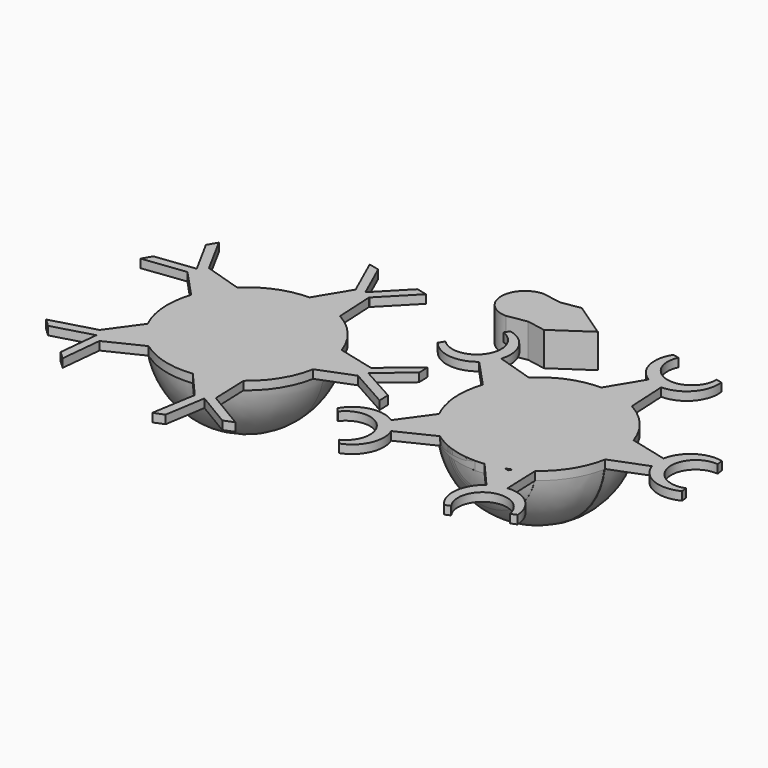
from build123d import *

# Parameters (mm, degrees)
F3_DEPTH = 1.27
F4_ANGLE = 180
F5_ANGLE = 180
F6_DEPTH = 5.08


# Not quite as in the source:
# - a feature names something its author has since deleted; it is built from what else it names


with BuildPart() as f3:
    # F0 (on Top) → F3 (new body)
    with BuildSketch(Plane.XY):
        with BuildLine():
            Line((4.8936784242, -7.1238775551), (4.5592080627, -7.6555667928))
            Line((4.5592080627, -7.6555667928), (3.9454245804, -7.5005655384))
            ThreePointArc((3.9454245804, -7.5005655384), (2.6783186026, -7.8645703011), (1.3787031683, -8.086057883))
            Line((1.3787031683, -8.086057883), (4.9129540048, -12.1410587354))
            Line((4.9129540048, -12.1410587354), (4.9601170844, -12.1951710033))
            Line((4.9601170844, -12.1951710033), (6.1814893534, -11.7059845827))
            Line((6.1814893534, -11.7059845827), (7.3584312348, -11.2345935081))
            Line((7.3584312348, -11.2345935081), (7.1565504338, -5.792935627))
            ThreePointArc((7.1565504338, -5.792935627), (6.061960316, -6.5210520939), (4.8936784242, -7.1238775551))
        make_face()
        with BuildLine():
            ThreePointArc((1.3787031683, -8.086057883), (2.6783186026, -7.8645703011), (3.9454245804, -7.5005655384))
            ThreePointArc((3.9454245804, -7.5005655384), (4.1864101627, -7.4136951085), (4.4254683384, -7.3216532098))
            ThreePointArc((4.4254683384, -7.3216532098), (4.6606303031, -7.2252675178), (4.8936784242, -7.1238775551))
            ThreePointArc((4.8936784242, -7.1238775551), (6.061960316, -6.5210520939), (7.1565504338, -5.792935627))
            Line((7.1565504338, -5.792935627), (7.1556255471, -5.7680054855))
            ThreePointArc((7.1556255471, -5.7680054855), (10.1274372954, -2.5017266103), (11.7022892851, 1.6238138354))
            Line((11.7022892851, 1.6238138354), (11.7389820542, 1.6381275484))
            ThreePointArc((11.7389820542, 1.6381275484), (11.8913668028, 4.6083597915), (11.3018507931, 7.5234878441))
            Line((11.3018507931, 7.5234878441), (11.2645029558, 7.5329194463))
            ThreePointArc((11.2645029558, 7.5329194463), (9.1157339139, 11.3612670795), (5.7241812928, 14.1488869988))
            Line((5.7241812928, 14.1488869988), (5.7231708963, 14.1682476177))
            ThreePointArc((5.7231708963, 14.1682476177), (2.9312146583, 15.2592925332), (-0.0448824936, 15.6174047842))
            Line((-0.0448824936, 15.6174047842), (0, -8.1622908183))
            ThreePointArc((0, -8.1622908183), (0.6889378263, -8.1423144191), (1.3755606611, -8.0824523468))
            Line((1.3755606611, -8.0824523468), (1.3787031683, -8.086057883))
        make_face()
        with BuildLine():
            ThreePointArc((0, -8.1622908183), (0.6904591534, -8.1442051837), (1.3787031683, -8.086057883))
            Line((1.3787031683, -8.086057883), (1.3755606611, -8.0824523468))
            ThreePointArc((1.3755606611, -8.0824523468), (0.6889378263, -8.1423144191), (0, -8.1622908183))
        make_face()
        with BuildLine():
            Line((7.1556255471, -5.7680054855), (7.1565504338, -5.792935627))
            ThreePointArc((7.1565504338, -5.792935627), (10.1544844582, -2.5132081517), (11.7389820542, 1.6381275484))
            Line((11.7389820542, 1.6381275484), (11.7022892851, 1.6238138354))
            ThreePointArc((11.7022892851, 1.6238138354), (10.1274372954, -2.5017266103), (7.1556255471, -5.7680054855))
        make_face()
        with BuildLine():
            Line((4.9601170844, -12.1951710033), (4.9129540048, -12.1410587354))
            ThreePointArc((4.9129540048, -12.1410587354), (2.9744543706, -15.5193953097), (4.1887523177, -19.2202626859))
            Line((4.1887523177, -19.2202626859), (5.0008226603, -18.8854850019))
            ThreePointArc((5.0008226603, -18.8854850019), (6.5893352056, -13.3433475455), (11.622070306, -16.1558619191))
            Line((11.622070306, -16.1558619191), (12.518363314, -15.7863632665))
            ThreePointArc((12.518363314, -15.7863632665), (10.9032070899, -12.4167602553), (7.3584312348, -11.2345935081))
            Line((7.3584312348, -11.2345935081), (6.1814893534, -11.7059845827))
            Line((6.1814893534, -11.7059845827), (4.9601170844, -12.1951710033))
        make_face()
        with BuildLine():
            ThreePointArc((-7.0516919086, -5.8454424545), (-3.7112715178, -7.5682384641), (0, -8.1622908183))
            Line((0, -8.1622908183), (-0.0448824936, 15.6174047842))
            ThreePointArc((-0.0448824936, 15.6174047842), (-4.4734734608, 14.743838405), (-8.2573042209, 12.2825052394))
            Line((-8.2573042209, 12.2825052394), (-13.7991155098, 14.0226887463))
            Line((-13.7991155098, 14.0226887463), (-13.8825975476, 14.0489029311))
            Line((-13.8825975476, 14.0489029311), (-14.5983996738, 12.9110314466))
            Line((-14.5983996738, 12.9110314466), (-15.319207147, 11.7652032356))
            Line((-15.319207147, 11.7652032356), (-11.2936160838, 7.4456261961))
            ThreePointArc((-11.2936160838, 7.4456261961), (-11.8627160209, 2.9241962242), (-10.6891807971, -1.4792136827))
            Line((-10.6891807971, -1.4792136827), (-14.1287515965, -6.2587273525))
            Line((-14.1287515965, -6.2587273525), (-14.1557744366, -6.2962773961))
            Line((-14.1557744366, -6.2962773961), (-13.2794303468, -7.3470839927))
            Line((-13.2794303468, -7.3470839927), (-12.3756340088, -8.4308080287))
            Line((-12.3756340088, -8.4308080287), (-7.0516919086, -5.8454424545))
        make_face()
        with BuildLine():
            ThreePointArc((11.3018507931, 7.5234878441), (11.8913668028, 4.6083597915), (11.7389820542, 1.6381275484))
            Line((11.7389820542, 1.6381275484), (17.0952796063, 3.7275993392))
            Line((17.0952796063, 3.7275993392), (17.0191165937, 4.8661190757))
            Line((17.0191165937, 4.8661190757), (16.936538316, 6.1005371469))
            Line((16.936538316, 6.1005371469), (11.3018507931, 7.5234878441))
        make_face()
        with BuildLine():
            Line((3.0023803732, 20.6531485623), (-0.0448824936, 15.6174047842))
            ThreePointArc((-0.0448824936, 15.6174047842), (2.9312146583, 15.2592925332), (5.7231708963, 14.1682476177))
            Line((5.7231708963, 14.1682476177), (5.4165524673, 20.0434878046))
            Line((5.4165524673, 20.0434878046), (5.4515073631, 20.0616481273))
            ThreePointArc((5.4515073631, 20.0616481273), (9.0104590154, 21.6991770677), (10.1547438103, 25.4459423662))
            Line((10.1547438103, 25.4459423662), (9.2975141381, 25.6374929551))
            ThreePointArc((9.2975141381, 25.6374929551), (4.8174413872, 22.0087730928), (2.308058113, 27.1993082555))
            Line((2.308058113, 27.1993082555), (1.3619221427, 27.4107252283))
            ThreePointArc((1.3619221427, 27.4107252283), (0.7522557785, 23.7240924821), (2.9779031767, 20.7225182718))
            Line((2.9779031767, 20.7225182718), (3.0023803732, 20.6531485623))
        make_face()
        with BuildLine():
            Line((17.0191165937, 4.8661190757), (17.0952796063, 3.7275993392))
            Line((17.0952796063, 3.7275993392), (17.1615459763, 3.5500786447))
            ThreePointArc((17.1615459763, 3.5500786447), (19.9175529921, 0.7658259222), (23.8297291445, 0.9720191488))
            Line((23.8297291445, 0.9720191488), (23.7165380041, 1.8430657059))
            ThreePointArc((23.7165380041, 1.8430657059), (18.7743816021, 4.8118617231), (22.7936295654, 8.9451782489))
            Line((22.7936295654, 8.9451782489), (22.6686989745, 9.9065641017))
            ThreePointArc((22.6686989745, 9.9065641017), (18.99587921, 9.2185604251), (16.936538316, 6.1005371469))
            Line((16.936538316, 6.1005371469), (17.0191165937, 4.8661190757))
        make_face()
        with BuildLine():
            Line((11.2645029558, 7.5329194463), (11.3018507931, 7.5234878441))
            ThreePointArc((11.3018507931, 7.5234878441), (9.1402278714, 11.3728743462), (5.7231708963, 14.1682476177))
            Line((5.7231708963, 14.1682476177), (5.7241812928, 14.1488869988))
            ThreePointArc((5.7241812928, 14.1488869988), (9.1157339139, 11.3612670795), (11.2645029558, 7.5329194463))
        make_face()
        with BuildLine():
            ThreePointArc((-15.1732003523, -14.7170731798), (-12.4419573589, -12.1669230289), (-12.3756340088, -8.4308080287))
            Line((-12.3756340088, -8.4308080287), (-13.2794303468, -7.3470839927))
            Line((-13.2794303468, -7.3470839927), (-14.1557744366, -6.2962773961))
            Line((-14.1557744366, -6.2962773961), (-14.1287515965, -6.2587273525))
            ThreePointArc((-14.1287515965, -6.2587273525), (-17.8700326747, -5.5513592404), (-20.9440362427, -7.7981471289))
            Line((-20.9440362427, -7.7981471289), (-20.3814259743, -8.4726869905))
            ThreePointArc((-20.3814259743, -8.4726869905), (-14.6179304287, -8.3285384937), (-15.7941609063, -13.9725744216))
            Line((-15.7941609063, -13.9725744216), (-15.1732003523, -14.7170731798))
        make_face()
        with BuildLine():
            Line((-13.8825975476, 14.0489029311), (-13.7991155098, 14.0226887463))
            ThreePointArc((-13.7991155098, 14.0226887463), (-14.2148294559, 17.8410690858), (-17.3031498513, 20.1247336053))
            Line((-17.3031498513, 20.1247336053), (-17.7763383415, 19.3847153679))
            ThreePointArc((-17.7763383415, 19.3847153679), (-15.8987321883, 13.9337287759), (-21.6344994058, 13.3509474106))
            Line((-21.6344994058, 13.3509474106), (-22.1567639352, 12.5341792845))
            ThreePointArc((-22.1567639352, 12.5341792845), (-18.9009805253, 10.7003776406), (-15.319207147, 11.7652032356))
            Line((-15.319207147, 11.7652032356), (-14.5983996738, 12.9110314466))
            Line((-14.5983996738, 12.9110314466), (-13.8825975476, 14.0489029311))
        make_face()
    extrude(amount=-F3_DEPTH)

    # F0 (on Top) → F5 (revolve)
    with BuildSketch(Plane.XY):
        with BuildLine():
            ThreePointArc((1.3787031683, -8.086057883), (2.6783186026, -7.8645703011), (3.9454245804, -7.5005655384))
            ThreePointArc((3.9454245804, -7.5005655384), (4.1864101627, -7.4136951085), (4.4254683384, -7.3216532098))
            ThreePointArc((4.4254683384, -7.3216532098), (4.6606303031, -7.2252675178), (4.8936784242, -7.1238775551))
            ThreePointArc((4.8936784242, -7.1238775551), (6.061960316, -6.5210520939), (7.1565504338, -5.792935627))
            Line((7.1565504338, -5.792935627), (7.1556255471, -5.7680054855))
            ThreePointArc((7.1556255471, -5.7680054855), (10.1274372954, -2.5017266103), (11.7022892851, 1.6238138354))
            Line((11.7022892851, 1.6238138354), (11.7389820542, 1.6381275484))
            ThreePointArc((11.7389820542, 1.6381275484), (11.8913668028, 4.6083597915), (11.3018507931, 7.5234878441))
            Line((11.3018507931, 7.5234878441), (11.2645029558, 7.5329194463))
            ThreePointArc((11.2645029558, 7.5329194463), (9.1157339139, 11.3612670795), (5.7241812928, 14.1488869988))
            Line((5.7241812928, 14.1488869988), (5.7231708963, 14.1682476177))
            ThreePointArc((5.7231708963, 14.1682476177), (2.9312146583, 15.2592925332), (-0.0448824936, 15.6174047842))
            Line((-0.0448824936, 15.6174047842), (0, -8.1622908183))
            ThreePointArc((0, -8.1622908183), (0.6889378263, -8.1423144191), (1.3755606611, -8.0824523468))
            Line((1.3755606611, -8.0824523468), (1.3787031683, -8.086057883))
        make_face()
    revolve(axis=Axis((-0.0224412468, 3.7275569829, 0), (-0.0018874259, 0.9999982188, 0)), revolution_arc=F5_ANGLE)


with BuildPart() as f3b:
    # F1 (on Top) → F3, piece 2 (new body)
    with BuildSketch(Plane.XY):
        Polygon((-56.3787087709, 8.2594288565), (-55.6579012977, 9.4052570675), (-54.9553977499, 10.5219885294), (-58.118801564, 16.3542572409), (-58.943148782, 14.9484505672), (-55.9927480832, 9.5441184738), (-61.9329048645, 8.8191202889), (-62.7491450525, 7.4271389994), (-56.3328742423, 8.2102470658), align=None)
        Polygon((-54.9553977499, 10.5219885294), (-55.6579012977, 9.4052570675), (-56.3787087709, 8.2594288565), (-56.3328742423, 8.2102470658), (-56.2243428206, 8.2234933632), (-55.5830278484, 9.3171646319), (-54.917502783, 10.4521227636), align=None)
        with BuildLine():
            Line((-54.9420991715, 10.5431285521), (-54.9553977499, 10.5219885294))
            Line((-54.9553977499, 10.5219885294), (-54.917502783, 10.4521227636))
            Line((-54.917502783, 10.4521227636), (-55.5830278484, 9.3171646319))
            Line((-55.5830278484, 9.3171646319), (-56.2243428206, 8.2234933632))
            Line((-56.2243428206, 8.2234933632), (-56.3328742423, 8.2102470658))
            Line((-56.3328742423, 8.2102470658), (-52.3531177078, 3.9398518171))
            ThreePointArc((-52.3531177078, 3.9398518171), (-52.9222176448, -0.5815781548), (-51.748682421, -4.9849880617))
            Line((-51.748682421, -4.9849880617), (-55.2152760605, -9.8020517752))
            Line((-55.2152760605, -9.8020517752), (-55.1125047872, -9.9252827448))
            Line((-55.1125047872, -9.9252827448), (-54.3200248973, -10.6687635971))
            Line((-54.3200248973, -10.6687635971), (-53.3954023636, -11.5362167126))
            Line((-53.3954023636, -11.5362167126), (-53.4361407581, -11.9353771822))
            Line((-53.4361407581, -11.9353771822), (-53.4351356328, -11.9365824077))
            Line((-53.4351356328, -11.9365824077), (-48.1111935325, -9.3512168335))
            ThreePointArc((-48.1111935325, -9.3512168335), (-44.1100212189, -11.2700773262), (-39.6839409629, -11.5882267258))
            Line((-39.6839409629, -11.5882267258), (-36.0993845395, -15.7009453824))
            Line((-36.0993845395, -15.7009453824), (-34.8780122705, -15.2117589617))
            Line((-34.8780122705, -15.2117589617), (-33.7010703891, -14.7403678871))
            Line((-33.7010703891, -14.7403678871), (-33.9038760768, -9.2737798645))
            ThreePointArc((-33.9038760768, -9.2737798645), (-30.9320643285, -6.0075009893), (-29.3572123388, -1.8819605437))
            Line((-29.3572123388, -1.8819605437), (-24.1694101963, 0.1417818134))
            Line((-24.1694101963, 0.1417818134), (-24.2098127149, 1.4082695954))
            Line((-24.2098127149, 1.4082695954), (-24.2486760676, 2.6265095255))
            Line((-24.2486760676, 2.6265095255), (-29.7949986682, 4.0271450673))
            ThreePointArc((-29.7949986682, 4.0271450673), (-31.94376771, 7.8554927005), (-35.3353203311, 10.6431126198))
            Line((-35.3353203311, 10.6431126198), (-35.6406571337, 16.4937950435))
            Line((-35.6406571337, 16.4937950435), (-36.8956075562, 16.78751286))
            Line((-36.8956075562, 16.78751286), (-38.103772586, 17.0702806795))
            Line((-38.103772586, 17.0702806795), (-41.1043841175, 12.1116304052))
            ThreePointArc((-41.1043841175, 12.1116304052), (-45.5329750847, 11.2380640259), (-49.3168058449, 8.7767308603))
            Line((-49.3168058449, 8.7767308603), (-54.9420991715, 10.5431285521))
        make_face()
        with BuildLine():
            ThreePointArc((-41.0595016239, -11.5532537391), (-52.8345593495, 0.1996003715), (-41.1039507221, 11.9968197649))
            ThreePointArc((-41.1039507221, 11.9968197649), (-32.7489936146, 8.5637632842), (-29.2844229247, 0.2218249602))
            ThreePointArc((-29.2844229247, 0.2218249602), (-32.7332636267, -8.1044130371), (-41.0595016239, -11.5532537391))
        make_face(mode=Mode.SUBTRACT)
        Polygon((-38.130080717, 17.0764380278), (-38.103772586, 17.0702806795), (-38.0571212508, 17.1473741833), (-36.8614739914, 16.8454324883), (-35.6429491567, 16.5377134256), (-35.6406571337, 16.4937950435), (-35.6145321613, 16.4876805631), (-30.9241749346, 21.2922673672), (-32.5109685697, 21.6636522071), (-36.8000731159, 17.2460451794), (-39.2505349895, 22.7055617844), (-40.8217233269, 23.0732942458), align=None)
        Polygon((-38.0571212508, 17.1473741833), (-38.103772586, 17.0702806795), (-36.8956075562, 16.78751286), (-35.6406571337, 16.4937950435), (-35.6429491567, 16.5377134256), (-36.8614739914, 16.8454324883), align=None)
        Polygon((-54.3200248973, -10.6687635971), (-55.1125047872, -9.9252827448), (-54.3389319707, -10.8528583718), (-53.4361407581, -11.9353771822), (-53.3954023636, -11.5362167126), align=None)
        Polygon((-54.3389319707, -10.8528583718), (-55.1125047872, -9.9252827448), (-55.2795525849, -9.7685635137), (-61.7438144982, -11.5842791274), (-60.5553033196, -12.6993046509), (-54.6320263092, -11.018097014), (-55.2396223782, -16.9714080231), (-54.0627995945, -18.0754678452), (-53.4361407581, -11.9353771822), align=None)
        Polygon((-24.2502375982, 2.6754584394), (-24.2486760676, 2.6265095255), (-24.1229633079, 2.5947627679), (-24.0403850302, 1.3603446967), (-23.9642220177, 0.2218249602), (-24.1694101963, 0.1417818134), (-24.1678617637, 0.0932434773), (-18.3130335063, -3.1937751337), (-18.3649957114, -1.5649287109), (-23.7421783728, 1.4346673093), (-19.1029164872, 5.2146585937), (-19.1543676708, 6.8274861514), align=None)
        Polygon((-24.1229633079, 2.5947627679), (-24.2486760676, 2.6265095255), (-24.2098127149, 1.4082695954), (-24.1694101963, 0.1417818134), (-23.9642220177, 0.2218249602), (-24.0403850302, 1.3603446967), align=None)
        Polygon((-34.8780122705, -15.2117589617), (-36.0993845395, -15.7009453824), (-37.1857024729, -22.3269108683), (-35.6728596299, -21.7209840806), (-34.6932661689, -15.6421629523), (-29.5545152372, -18.7088099512), (-28.0565504239, -18.1088421413), (-33.7010703891, -14.7403678871), align=None)
        with BuildLine():
            Line((-41.0595016239, -11.5532537391), (-41.1039507221, 11.9968197649))
            ThreePointArc((-41.1039507221, 11.9968197649), (-52.8345593495, 0.1996003715), (-41.0595016239, -11.5532537391))
        make_face()
        with BuildLine():
            ThreePointArc((-29.2844229247, 0.2218249602), (-32.7489936146, 8.5637632842), (-41.1039507221, 11.9968197649))
            Line((-41.1039507221, 11.9968197649), (-41.0595016239, -11.5532537391))
            ThreePointArc((-41.0595016239, -11.5532537391), (-32.7332636267, -8.1044130371), (-29.2844229247, 0.2218249602))
        make_face()
    extrude(amount=-F3_DEPTH)

    # F1 (on Top) → F4 (revolve)
    with BuildSketch(Plane.XY):
        with BuildLine():
            ThreePointArc((-29.2844229247, 0.2218249602), (-32.7489936146, 8.5637632842), (-41.1039507221, 11.9968197649))
            Line((-41.1039507221, 11.9968197649), (-41.0595016239, -11.5532537391))
            ThreePointArc((-41.0595016239, -11.5532537391), (-32.7332636267, -8.1044130371), (-29.2844229247, 0.2218249602))
        make_face()
    revolve(axis=Axis((-41.081726173, 0.2217830129, 0), (-0.0018874259, 0.9999982188, 0)), revolution_arc=F4_ANGLE)


with BuildPart() as f6:
    # F2 (on Top) → F6 (new body)
    with BuildSketch(Plane.XY):
        Polygon((-17.3071837053, 29.5017343043), (-20.1507005841, 29.9917282594), (-20.1507005841, 22.8599924594), (-17.2187019579, 23.365233562), (-14.4636668265, 22.8599924594), (-14.4636668265, 29.9917282594), align=None)
        Polygon((-9.2094540596, 26.4270743384), (-14.4636668265, 29.9917282594), (-14.4636668265, 22.8599924594), align=None)
        with BuildLine():
            Line((-20.1507005841, 22.8599924594), (-20.1507005841, 29.9917282594))
            ThreePointArc((-20.1507005841, 29.9917282594), (-23.7165684841, 26.4258603594), (-20.1507005841, 22.8599924594))
        make_face()
    extrude(amount=-F6_DEPTH)


solid = Compound([f3.part, f3b.part, f6.part])
